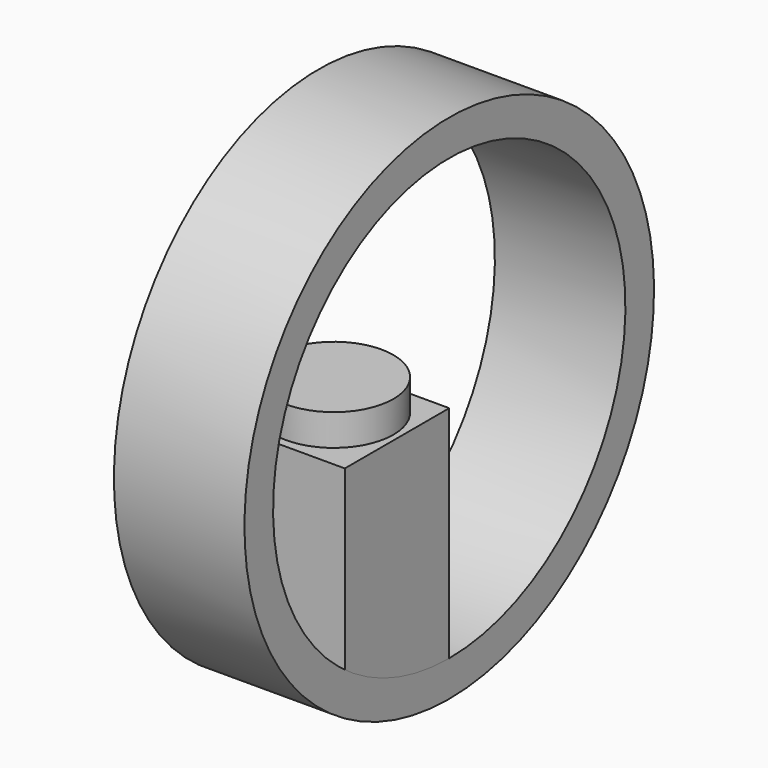
from build123d import *

# Parameters (mm, degrees)
F1_R     = 12.0249392967
F2_DEPTH = 50.8
F0_W     = 26.346960105
F0_H     = 26.346960105
F3_DEPTH = 44.45


# Not quite as in the source:
# - the program builds the solid bodies; features that only make, move or delete a surface that nothing else refers to are left out


with BuildPart() as f2:
    # F1 (on Top) → F2 (new body)
    with BuildSketch(Plane.XY):
        with Locations((-15.5347883701, 21.2581306696)):
            Circle(F1_R)
    extrude(amount=F2_DEPTH)

    # F0 (on Top) → F3 (join)
    with BuildSketch(Plane.XY):
        with Locations((-15.4747529887, 20.6551658921)):
            Rectangle(F0_W, F0_H)
    extrude(amount=F3_DEPTH)


with BuildPart() as f5:
    # F0 (on Top) → F5 (revolve)
    with BuildSketch(Plane.XY):
        with Locations((-15.4747529887, 20.6551658921)):
            Rectangle(F0_W, F0_H)
    revolve(axis=Axis((-15.4747529887, 33.8286459446, 44.45), (1, 0, 0)))


solid = Compound([f2.part, f5.part])
